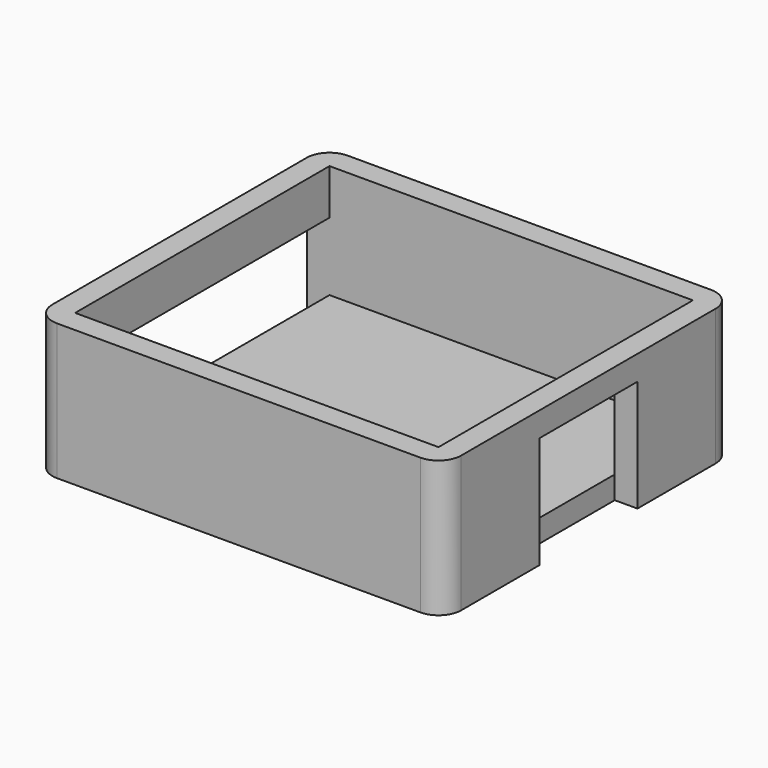
from build123d import *

# Parameters (mm, degrees)
F1_DEPTH = 19.05
F2_T     = 3.175
F3_W     = 17.145
F3_H     = 15.621
F4_DEPTH = 3.175
F5_W     = 44.45
F5_H     = 12.7
F6_DEPTH = 3.175


# Not quite as in the source:
# - a shell that OpenCascade refuses in one call is made with other operations: the cavity is built on its own and cut out


with BuildPart() as f1:
    # F0 (on Top) → F1 (new body)
    with BuildSketch(Plane.XY):
        with BuildLine():
            Line((-25.4, -25.4), (25.4, -25.4))
            ThreePointArc((25.4, -25.4), (27.6450640303, -24.4700640303), (28.575, -22.225))
            Line((28.575, -22.225), (28.575, 22.225))
            ThreePointArc((28.575, 22.225), (27.6450640303, 24.4700640303), (25.4, 25.4))
            Line((25.4, 25.4), (-25.4, 25.4))
            ThreePointArc((-25.4, 25.4), (-27.6450640303, 24.4700640303), (-28.575, 22.225))
            Line((-28.575, 22.225), (-28.575, -22.225))
            ThreePointArc((-28.575, -22.225), (-27.6450640303, -24.4700640303), (-25.4, -25.4))
        make_face()
    extrude(amount=F1_DEPTH)

    # F2: shell of thickness 3.175, made by hand


with BuildPart() as f2_core1:
    # F2_t2: copy of F1
    add(f1.part)

    # the walls: a layer under each face that stays
    f2_faces = [f2_core1.faces().sort_by_distance(p)[0] for p in [
        (0, -25.4, 9.525),
        (28.575, 0, 9.525),
        (0, 25.4, 9.525),
        (-28.575, 0, 9.525),
        (0, 0, 0),
    ]]
    thicken(f2_faces, amount=-F2_T, mode=Mode.SUBTRACT)


with BuildPart() as f1_1:
    add(f1.part)

    # what is left inside the walls is the cavity
    f2_cavity = [f2_core1.part.solids().sort_by_distance(p)[0] for p in [
        (0, -7.408333, 3.20675),
    ]]
    add(f2_cavity, mode=Mode.SUBTRACT)

    # F3 (on face) → F4 (cut)
    with BuildSketch(Plane.YZ.offset(28.575)):
        with Locations((0, 7.8105)):
            Rectangle(F3_W, F3_H)
    extrude(amount=-F4_DEPTH, mode=Mode.SUBTRACT)

    # F5 (on face) → F6 (cut)
    with BuildSketch(Plane(origin=(-28.575, 0, 0), x_dir=(0, -1, 0), z_dir=(-1, 0, 0))):
        with Locations((0, 6.35)):
            Rectangle(F5_W, F5_H)
    extrude(amount=-F6_DEPTH, mode=Mode.SUBTRACT)


solid = f1_1.part
